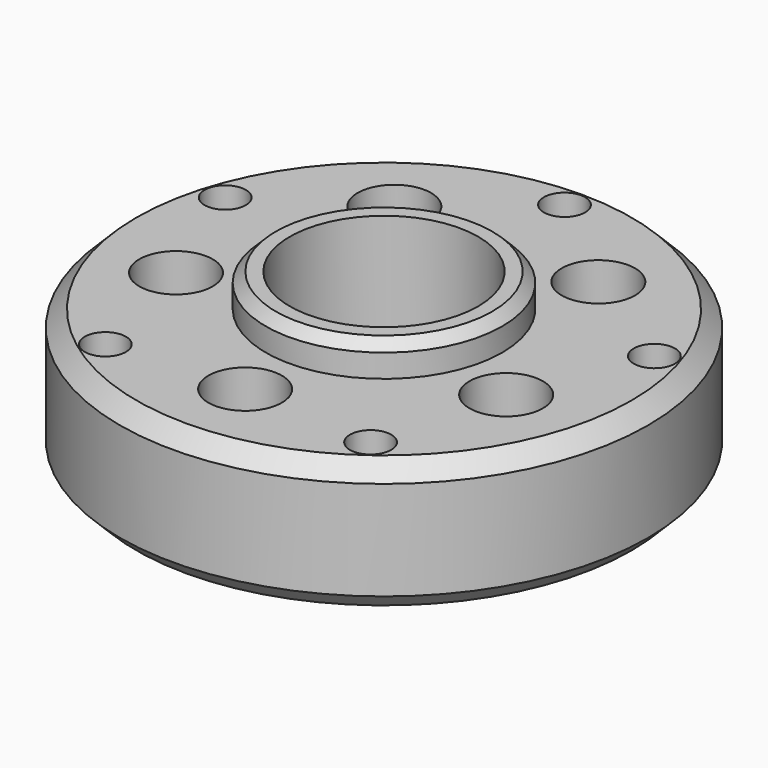
from build123d import *

# Parameters (mm, degrees)
F0_R             = 80
F1_DEPTH         = 20
F2_R             = 35.8
F3_DEPTH         = 10
F6_R             = 28.55
F7_DEPTH         = 50.001
F9_D             = 15.5
F9_CBORE_D       = 22.25
F9_CBORE_DEPTH   = 14
F9_COPIES_COUNT  = 5
F10_D            = 12.5
F10_COPIES_COUNT = 5
F11_SIZE         = 5
F12_SIZE         = 3


# Not quite as in the source:
# - a pattern or mirror of a feature is missing from the dataset's text; its kind, count and spacing are read off the source's solid
# - the program builds the solid bodies; features that only make, move or delete a surface that nothing else refers to are left out


with BuildPart() as f1:
    # F0 (on Top) → F1 (new body, symmetric)
    with BuildSketch(Plane.XY):
        Circle(F0_R)
    extrude(amount=F1_DEPTH, both=True)

    # F2 (on face) → F3 (join)
    with BuildSketch(Plane.XY.offset(20)):
        Circle(F2_R)
    extrude(amount=F3_DEPTH)

    # F6 (on face) → F7 (cut, through all)
    with BuildSketch(Plane(origin=(0, 0, -20), x_dir=(1, 0, 0), z_dir=(0, 0, -1))):
        Circle(F6_R)
    extrude(amount=-F7_DEPTH, mode=Mode.SUBTRACT)

    # F9 (through all)
    with Locations(Plane.XY.offset(20)):
        with Locations((-30.9016994375, 42.5325404176)):
            f9 = CounterBoreHole(F9_D / 2, F9_CBORE_D / 2, F9_CBORE_DEPTH)

    # F9_copies: F9 ×5 about axis
    f9_copies_axis = Axis((0, 0, 0), (0, 0, 1))
    for i in range(1, F9_COPIES_COUNT):
        add(f9.rotate(f9_copies_axis, i * 360 / F9_COPIES_COUNT), mode=Mode.SUBTRACT)

    # F10 (through all)
    with Locations(Plane.XY.offset(20)):
        with Locations((0, 68.3450445755)):
            f10 = Hole(F10_D / 2)

    # F10_copies: F10 ×5 about axis
    f10_copies_axis = Axis((0, 0, 0), (0, 0, 1))
    for i in range(1, F10_COPIES_COUNT):
        add(f10.rotate(f10_copies_axis, i * 360 / F10_COPIES_COUNT), mode=Mode.SUBTRACT)

    # F11
    f11_edges = [f1.edges().sort_by_distance(p)[0] for p in [
        (-80, 0, 20),
        (-28.55, 0, -20),
        (-80, 0, -20),
    ]]
    chamfer(f11_edges, length=F11_SIZE)

    # F12
    f12_edges = [f1.edges().sort_by_distance(p)[0] for p in [
        (-35.8, 0, 30),
    ]]
    chamfer(f12_edges, length=F12_SIZE)


solid = f1.part
